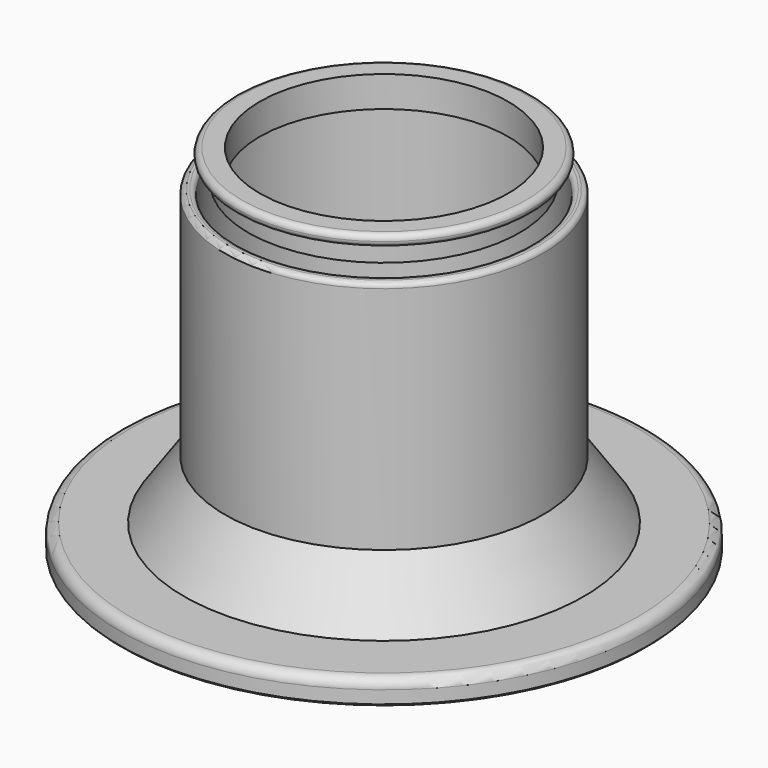
from build123d import *

# Parameters (mm, degrees)
F6_R     = 2.54
F7_R     = 5.4631705107
F8_DEPTH = 82.551
F9_SIZE  = 0.5
F10_R    = 1.27
F11_R    = 1.27
F13_R    = 1.5
F14_R    = 1.49999


# Not quite as in the source:
# - a fillet or chamfer is up to 0.001 mm smaller than in the source, because OpenCascade refuses the exact size


with BuildPart() as f5:
    # F2 (on Front) → F5 (revolve)
    with BuildSketch(Plane.XZ):
        Polygon((-51.875, 6.35), (-68.5, 6.35), (-68.5, 0), (0, 0), (0, 6.35), (-38.1213697813, 6.35), (-38.1213697813, 82.55), (-41.2963697813, 82.55), (-41.2963697813, 21.59), align=None)
    revolve(axis=Axis((0, 0, 3.175), (0, 0, 1)))

    # F6
    f6_edges = [f5.edges().sort_by_distance(p)[0] for p in [
        (68.5, 0, 6.35),
    ]]
    fillet(f6_edges, radius=F6_R)

    # F7 (on Top) → F8 (cut, through all)
    with BuildSketch(Plane.XY):
        Circle(F7_R)
    extrude(amount=F8_DEPTH, mode=Mode.SUBTRACT)

    # F9
    f9_edges = [f5.edges().sort_by_distance(p)[0] for p in [
        (68.5, 0, 0),
    ]]
    chamfer(f9_edges, length=F9_SIZE)

    # F10
    f10_edges = [f5.edges().sort_by_distance(p)[0] for p in [
        (38.12137, 0, 82.55),
    ]]
    fillet(f10_edges, radius=F10_R)

    # F11
    f11_edges = [f5.edges().sort_by_distance(p)[0] for p in [
        (41.29637, 0, 82.55),
    ]]
    fillet(f11_edges, radius=F11_R)


with BuildPart() as f12:
    # F4 (on Front) → F12 (revolve)
    with BuildSketch(Plane.XZ):
        Polygon((-35.25, 89.0617567301), (-35.25, 84.0617567301), (-32.25, 84.0617567301), (-32.25, 92.0617567301), (-38.425, 92.0617567301), (-38.425, 89.0617567301), align=None)
    revolve(axis=Axis((0, 0, 41.1046370864), (0, 0, 1)))

    # F13
    f13_edges = [f12.edges().sort_by_distance(p)[0] for p in [
        (38.425, 0, 92.061757),
    ]]
    fillet(f13_edges, radius=F13_R)

    # F14 (radius 1.5 in the source; OpenCascade refuses exactly that, so slightly less here)
    f14_edges = [f12.edges().sort_by_distance(p)[0] for p in [
        (38.425, 0, 89.061757),
        (-38.425, 0, 89.811757),
        (38.425, 0, 90.561757),
    ]]
    fillet(f14_edges, radius=F14_R)


solid = Compound([f5.part, f12.part])
